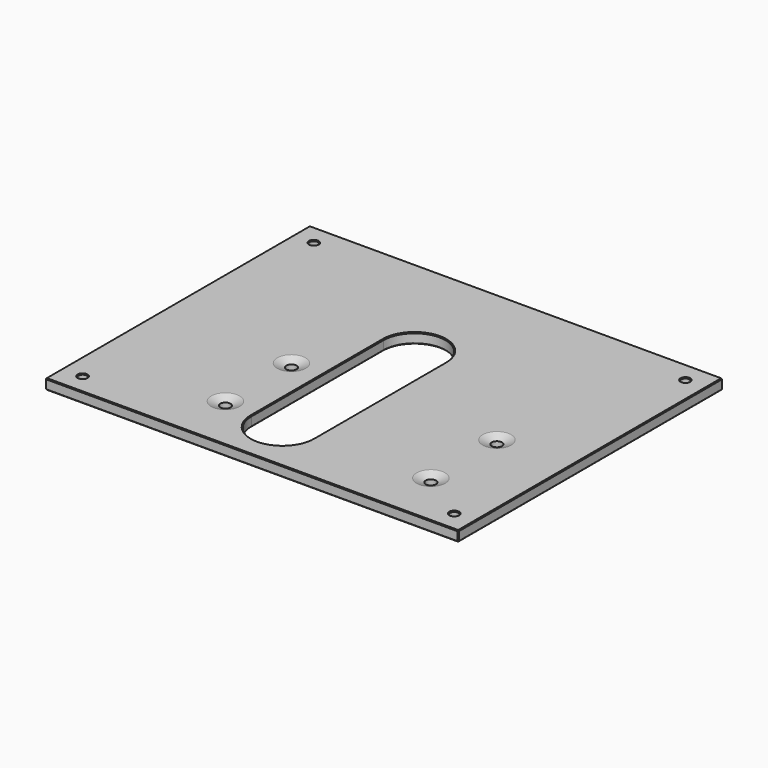
from build123d import *

# Parameters (mm, degrees)
F0_W     = 254
F0_H     = 203.2
F0_R     = 2.54
F0_R_2   = 3.175
F1_DEPTH = 6.35
F2_SIZE  = 0.508


# Not quite as in the source:
# - a fillet or chamfer that OpenCascade refuses, or shapes differently, is made with other operations: its cross-section is extruded or revolved along the edge and cut away or added


with BuildPart() as f1:
    # F0 (on Top) → F1 (new body)
    with BuildSketch(Plane.XY):
        with Locations((14.533196536, 0)):
            Rectangle(F0_W, F0_H)
        with Locations((-99.766803464, -88.9)):
            Circle(F0_R, mode=Mode.SUBTRACT)
        with Locations((-29.9168042839, -66.4009973407)):
            Circle(F0_R_2, mode=Mode.SUBTRACT)
        with Locations((-29.9168042839, -15.6009973407)):
            Circle(F0_R_2, mode=Mode.SUBTRACT)
        with BuildLine():
            ThreePointArc((27.2331968829, -70.1908171177), (8.1831968829, -89.2408171177), (-10.8668031171, -70.1908171177))
            Line((-10.8668031171, -70.1908171177), (-10.8668031171, 31.4091828823))
            ThreePointArc((-10.8668031171, 31.4091828823), (8.1831968829, 50.4591828823), (27.2331968829, 31.4091828823))
            Line((27.2331968829, 31.4091828823), (27.2331968829, -70.1908171177))
        make_face(mode=Mode.SUBTRACT)
        with Locations((128.833196536, -88.9)):
            Circle(F0_R, mode=Mode.SUBTRACT)
        with Locations((97.0831957161, -67.1428190649)):
            Circle(F0_R_2, mode=Mode.SUBTRACT)
        with Locations((97.0831957161, -16.3428190649)):
            Circle(F0_R_2, mode=Mode.SUBTRACT)
        with Locations((-99.766803464, 88.9)):
            Circle(F0_R, mode=Mode.SUBTRACT)
        with Locations((128.833196536, 88.9)):
            Circle(F0_R, mode=Mode.SUBTRACT)
    extrude(amount=F1_DEPTH)

    # F2
    f2_edges = [f1.edges().sort_by_distance(p)[0] for p in [
        (14.533197, -101.6, 6.35),
        (141.533197, 0, 6.35),
        (14.533197, 101.6, 6.35),
        (-112.466803, 0, 6.35),
        (-102.306803, -88.9, 6.35),
        (-33.091804, -66.400997, 6.35),
        (-33.091804, -15.600997, 6.35),
        (8.183197, 50.459183, 6.35),
        (27.233197, -19.390817, 6.35),
        (8.183197, -89.240817, 6.35),
        (-10.866803, -19.390817, 6.35),
        (126.293197, -88.9, 6.35),
        (93.908196, -67.142819, 6.35),
        (93.908196, -16.342819, 6.35),
        (-102.306803, 88.9, 6.35),
        (126.293197, 88.9, 6.35),
        (14.533197, -101.6, 0),
        (141.533197, 0, 0),
        (14.533197, 101.6, 0),
        (-112.466803, 0, 0),
        (-102.306803, -88.9, 0),
        (-33.091804, -66.400997, 0),
        (-33.091804, -15.600997, 0),
        (8.183197, 50.459183, 0),
        (27.233197, -19.390817, 0),
        (8.183197, -89.240817, 0),
        (-10.866803, -19.390817, 0),
        (126.293197, -88.9, 0),
        (93.908196, -67.142819, 0),
        (93.908196, -16.342819, 0),
        (-102.306803, 88.9, 0),
        (126.293197, 88.9, 0),
        (-112.466803, -101.6, 3.175),
        (-112.466803, 101.6, 3.175),
        (141.533197, -101.6, 3.175),
        (141.533197, 101.6, 3.175),
    ]]
    chamfer(f2_edges, length=F2_SIZE)

    # F3: chamfer of 5.08 on 4 edges, made by hand

    # F3_s1 → F3_t2 (revolve, cut)
    with BuildSketch(Plane.XZ.offset(66.4009973407)):
        Polygon((-21.1538042839, 6.35), (-29.8259067323, 2.7578975516), (-26.2338042839, 6.35), align=None)
    revolve(axis=Axis((-29.9168042839, -66.4009973407, 6.35), (0, 0, 1)), mode=Mode.SUBTRACT)

    # F3_s3 → F3_t4 (revolve, cut)
    with BuildSketch(Plane.XZ.offset(15.6009973407)):
        Polygon((-21.1538042839, 6.35), (-29.8259067323, 2.7578975516), (-26.2338042839, 6.35), align=None)
    revolve(axis=Axis((-29.9168042839, -15.6009973407, 6.35), (0, 0, 1)), mode=Mode.SUBTRACT)

    # F3_s5 → F3_t6 (revolve, cut)
    with BuildSketch(Plane.XZ.offset(67.1428190649)):
        Polygon((105.8461957161, 6.35), (97.1740932677, 2.7578975516), (100.7661957161, 6.35), align=None)
    revolve(axis=Axis((97.0831957161, -67.1428190649, 6.35), (0, 0, 1)), mode=Mode.SUBTRACT)

    # F3_s7 → F3_t8 (revolve, cut)
    with BuildSketch(Plane.XZ.offset(16.3428190649)):
        Polygon((105.8461957161, 6.35), (97.1740932677, 2.7578975516), (100.7661957161, 6.35), align=None)
    revolve(axis=Axis((97.0831957161, -16.3428190649, 6.35), (0, 0, 1)), mode=Mode.SUBTRACT)


solid = f1.part
